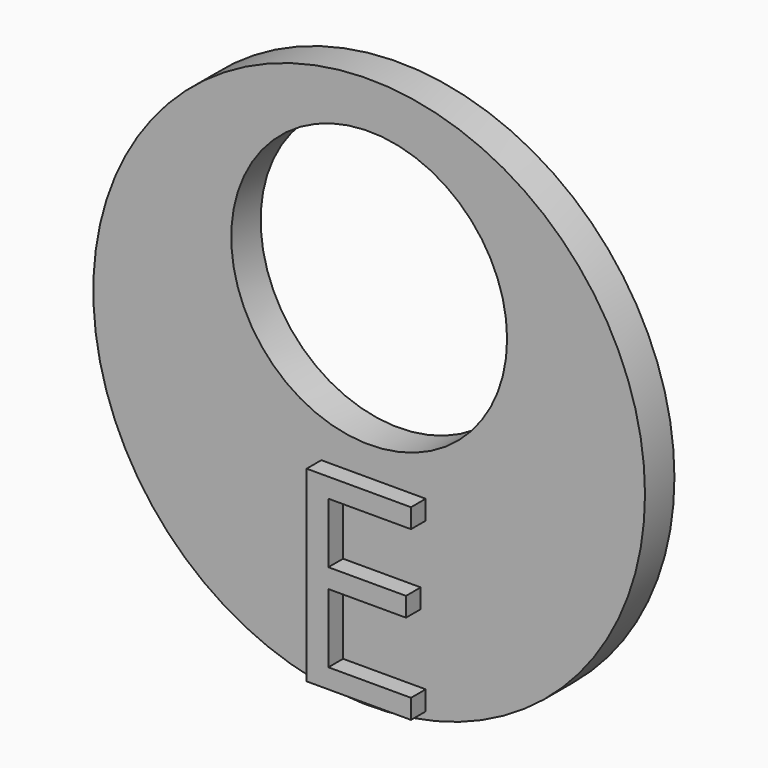
from build123d import *

# Parameters (mm, degrees)
F0_R         = 15
F0_R_2       = 7.5
F1_DEPTH     = 2
F2_TEXT_SIZE = 14.2618384401
F3_DEPTH     = 1


# Not quite as in the source:
# - Text() gives the source's letters only with a copy of the font that has no kerning and outlines rounded to 1/6400 em; it was checked with that copy


with BuildPart() as f1:
    # F0 (on Front) → F1 (new body)
    with BuildSketch(Plane.XZ):
        Circle(F0_R)
        with Locations((0, 5)):
            Circle(F0_R_2, mode=Mode.SUBTRACT)
    extrude(amount=F1_DEPTH)

    # F2 (on face) → F3 (join)
    with BuildSketch(Plane.XZ.offset(2)):
        with Locations((-4, -14.2685236769)):
            Text('E', F2_TEXT_SIZE, font='Open Sans', text_align=(TextAlign.LEFT, TextAlign.BOTTOM))
    extrude(amount=F3_DEPTH)


solid = f1.part
